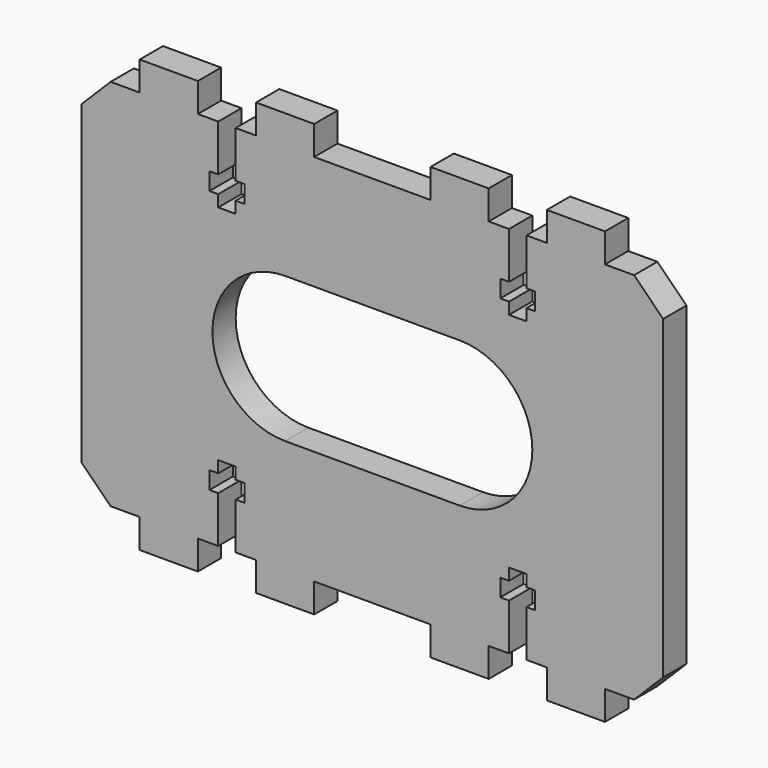
from build123d import *

# Parameters (mm, degrees)
F1_DEPTH = 5
F2_SIZE  = 5
F3_W     = 10
F3_H     = 5
F4_DEPTH = 5


# Not quite as in the source:
# - a pattern or mirror of a feature is missing from the dataset's text; its kind, count and spacing are read off the source's solid


with BuildPart() as f1:
    # F0 (on Front) → F1 (new body)
    with BuildSketch(Plane.XZ):
        Polygon((-26.5, 32.125), (-50, 32.125), (-50, -32.125), (-26.5, -32.125), (-26.5, -24.125), (-28, -24.125), (-28, -21.125), (-26.5, -21.125), (-26.5, -19.125), (-25, -19.125), (-23.5, -19.125), (-23.5, -21.125), (-22, -21.125), (-22, -24.125), (-23.5, -24.125), (-23.5, -32.125), (-1.5, -32.125), (-1.5, -24.125), (-3, -24.125), (-3, -21.125), (-1.5, -21.125), (-1.5, -19.125), (0, -19.125), (1.5, -19.125), (1.5, -21.125), (3, -21.125), (3, -24.125), (1.5, -24.125), (1.5, -32.125), (23.5, -32.125), (23.5, -24.125), (22, -24.125), (22, -21.125), (23.5, -21.125), (23.5, -19.125), (25, -19.125), (26.5, -19.125), (26.5, -21.125), (28, -21.125), (28, -24.125), (26.5, -24.125), (26.5, -32.125), (50, -32.125), (50, 32.125), (26.5, 32.125), (26.5, 24.125), (28, 24.125), (28, 21.125), (26.5, 21.125), (26.5, 19.125), (25, 19.125), (23.5, 19.125), (23.5, 21.125), (22, 21.125), (22, 24.125), (23.5, 24.125), (23.5, 32.125), (1.5, 32.125), (1.5, 24.125), (3, 24.125), (3, 21.125), (1.5, 21.125), (1.5, 19.125), (0, 19.125), (-1.5, 19.125), (-1.5, 21.125), (-3, 21.125), (-3, 24.125), (-1.5, 24.125), (-1.5, 32.125), (-23.5, 32.125), (-23.5, 24.125), (-22, 24.125), (-22, 21.125), (-23.5, 21.125), (-23.5, 19.125), (-25, 19.125), (-26.5, 19.125), (-26.5, 21.125), (-28, 21.125), (-28, 24.125), (-26.5, 24.125), align=None)
        with BuildLine():
            Line((15, -12.5), (-15, -12.5))
            ThreePointArc((-15, -12.5), (-27.5, 0), (-15, 12.5))
            Line((-15, 12.5), (15, 12.5))
            ThreePointArc((15, 12.5), (27.5, 0), (15, -12.5))
        make_face(mode=Mode.SUBTRACT)
        Polygon((1.5, 32.125), (-1.5, 32.125), (-1.5, 24.125), (-3, 24.125), (-3, 21.125), (-1.5, 21.125), (-1.5, 19.125), (0, 19.125), (1.5, 19.125), (1.5, 21.125), (3, 21.125), (3, 24.125), (1.5, 24.125), align=None)
        Polygon((-1.5, -24.125), (-1.5, -32.125), (1.5, -32.125), (1.5, -24.125), (3, -24.125), (3, -21.125), (1.5, -21.125), (1.5, -19.125), (0, -19.125), (-1.5, -19.125), (-1.5, -21.125), (-3, -21.125), (-3, -24.125), align=None)
    extrude(amount=F1_DEPTH)

    # F2
    f2_edges = [f1.edges().sort_by_distance(p)[0] for p in [
        (-50, -2.5, 32.125),
        (50, -2.5, 32.125),
        (-50, -2.5, -32.125),
        (50, -2.5, -32.125),
    ]]
    chamfer(f2_edges, length=F2_SIZE)

    # F3 (on face) → F4 (join)
    with BuildSketch(Plane(origin=(0, 0, -32.125), x_dir=(1, 0, 0), z_dir=(0, 0, -1))):
        with Locations((35, 2.5)):
            Rectangle(F3_W, F3_H)
        with Locations((15, 2.5)):
            Rectangle(F3_W, F3_H)
        with Locations((-15, 2.5)):
            Rectangle(F3_W, F3_H)
        with Locations((-35, 2.5)):
            Rectangle(F3_W, F3_H)
    f4 = extrude(amount=F4_DEPTH)

    # F4_copies: F4 across plane
    add(f4.mirror(Plane.XY))


solid = f1.part
